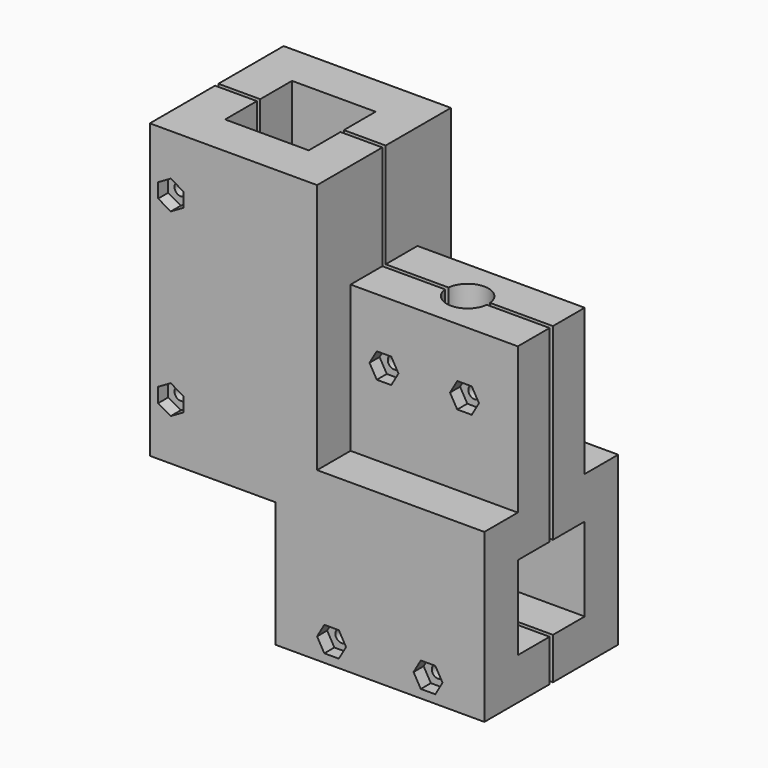
from build123d import *

# Parameters (mm, degrees)
F1_DEPTH        = 20
F2_W            = 50
F2_H            = 10
F3_DEPTH        = 10
F4_W            = 50
F4_H            = 10
F5_DEPTH        = 10
F6_W            = 50
F6_H            = 10
F7_DEPTH        = 30
F8_W            = 10
F8_H            = 10
F9_DEPTH        = 60
F10_W           = 10
F10_H           = 70
F11_DEPTH       = 30
F12_R           = 5
F13_DEPTH       = 15
F16_DEPTH       = 70
F17_T1_DEPTH    = 17.2150489639
F17_S1_T1_DEPTH = 10.5
F18_W           = 10
F18_H           = 70
F18_W_2         = 50
F18_H_2         = 10
F20_DEPTH       = 9.5
F19_W           = 10
F19_H           = 70
F19_W_2         = 50
F19_H_2         = 10
F21_DEPTH       = 9.5
F22_R           = 1.5
F23_DEPTH       = 3
F24_DEPTH       = 20
F25_R           = 1.5
F26_DEPTH       = 20
F27_R           = 1.5
F28_DEPTH       = 3
F29_DEPTH       = 10
F30_R           = 1.5
F31_DEPTH       = 10


# Not quite as in the source:
# - a fillet or chamfer that OpenCascade refuses, or shapes differently, is made with other operations: its cross-section is extruded or revolved along the edge and cut away or added


with BuildPart() as f1:
    # F0 (on Front) → F1 (new body)
    with BuildSketch(Plane.XZ):
        Polygon((-40, 89.1929870069), (-50, 89.1929870069), (-50, 19.1929870069), (0, 19.1929870069), (0, 64.1929870069), (-40, 64.1929870069), align=None)
    extrude(amount=F1_DEPTH)

    # F2 (on face) → F3 (join)
    with BuildSketch(Plane.XZ.offset(20)):
        with Locations((-25, 24.1929870069)):
            Rectangle(F2_W, F2_H)
    extrude(amount=F3_DEPTH)

    # F4 (on face) → F5 (join)
    with BuildSketch(Plane(origin=(0, 0, 0), x_dir=(-1, 0, 0), z_dir=(0, 1, 0))):
        with Locations((25, 24.1929870069)):
            Rectangle(F4_W, F4_H)
    extrude(amount=F5_DEPTH)

    # F6 (on face) → F7 (join)
    with BuildSketch(Plane(origin=(0, 0, 19.1929870069), x_dir=(1, 0, 0), z_dir=(0, 0, -1))):
        with Locations((-25, 25)):
            Rectangle(F6_W, F6_H)
        with Locations((-25, -5)):
            Rectangle(F6_W, F6_H)
    extrude(amount=F7_DEPTH)

    # F8 (on face) → F9 (join)
    with BuildSketch(Plane.XY.offset(29.1929870069)):
        with Locations((-45, 5)):
            Rectangle(F8_W, F8_H)
        with Locations((-45, -25)):
            Rectangle(F8_W, F8_H)
    extrude(amount=F9_DEPTH)

    # F10 (on face) → F11 (join)
    with BuildSketch(Plane(origin=(-50, 0, 0), x_dir=(0, -1, 0), z_dir=(-1, 0, 0))):
        with Locations((25, 54.1929870069)):
            Rectangle(F10_W, F10_H)
        with Locations((-5, 54.1929870069)):
            Rectangle(F10_W, F10_H)
    extrude(amount=F11_DEPTH)

    # F12 (on face) → F13 (cut)
    with BuildSketch(Plane.XY.offset(64.1929870069)):
        with Locations((-20, -10)):
            Circle(F12_R)
    extrude(amount=-F13_DEPTH, mode=Mode.SUBTRACT)

    # F15 (on face) + F14 (on face) → F16 (cut)
    with BuildSketch(Plane.XY.offset(64.1929870069)):
        with BuildLine():
            Line((0, -10.5), (0, -9.5))
            Line((0, -9.5), (-15.0250628145, -9.5))
            ThreePointArc((-15.0250628145, -9.5), (-15.0062696344, -9.7496861247), (-15, -10))
            ThreePointArc((-15, -10), (-15.0062696344, -10.2503138753), (-15.0250628145, -10.5))
            Line((-15.0250628145, -10.5), (0, -10.5))
        make_face()
        with BuildLine():
            Line((-15.0250628145, -9.5), (-24.9749371855, -9.5))
            ThreePointArc((-24.9749371855, -9.5), (-25, -10), (-24.9749371855, -10.5))
            Line((-24.9749371855, -10.5), (-15.0250628145, -10.5))
            ThreePointArc((-15.0250628145, -10.5), (-15.0062696344, -10.2503138753), (-15, -10))
            ThreePointArc((-15, -10), (-15.0062696344, -9.7496861247), (-15.0250628145, -9.5))
        make_face()
        with BuildLine():
            Line((-24.9749371855, -9.5), (-40, -9.5))
            Line((-40, -9.5), (-40, -10.5))
            Line((-40, -10.5), (-24.9749371855, -10.5))
            ThreePointArc((-24.9749371855, -10.5), (-25, -10), (-24.9749371855, -9.5))
        make_face()
    with BuildSketch(Plane.XY.offset(89.1929870069)):
        Polygon((-40, -10.5), (-40, -10), (-40, -9.5), (-50, -9.5), (-50, -10.5), align=None)
    extrude(amount=-F16_DEPTH, mode=Mode.SUBTRACT)

    # F17: chamfer of 3 on 1 edges, made by hand

    # F17_s2 → F17_t1 (cut)
    with BuildSketch(Plane.XZ.offset(2.7849510361)):
        Polygon((-47, 19.1929870069), (-50, 22.1929870069), (-50, 19.1929870069), align=None)
    extrude(amount=F17_T1_DEPTH, mode=Mode.SUBTRACT)

    # F17#s1: chamfer of 3 on 1 edges, made by hand

    # F17_s1_s2 → F17_s1_t1 (cut)
    with BuildSketch(Plane.XZ):
        Polygon((-50, 22.1929870069), (-47, 19.1929870069), (-50, 19.1929870069), align=None)
    extrude(amount=F17_S1_T1_DEPTH, mode=Mode.SUBTRACT)

    # F18 (on face) → F20 (join)
    with BuildSketch(Plane.XZ):
        with Locations((-75, 54.1929870069)):
            Rectangle(F18_W, F18_H)
        with Locations((-25, -5.8070129931)):
            Rectangle(F18_W_2, F18_H_2)
    extrude(amount=F20_DEPTH)

    # F19 (on face) → F21 (join)
    with BuildSketch(Plane(origin=(0, -20, 0), x_dir=(-1, 0, 0), z_dir=(0, 1, 0))):
        with Locations((75, 54.1929870069)):
            Rectangle(F19_W, F19_H)
        with Locations((25, -5.8070129931)):
            Rectangle(F19_W_2, F19_H_2)
    extrude(amount=F21_DEPTH)

    # F22 (on face) → F23 (cut)
    with BuildSketch(Plane.XZ.offset(30)):
        Polygon((-72, 77.4609361993), (-75, 79.1929870069), (-78, 77.4609361993), (-78, 73.9968345842), (-75, 72.2647837766), (-72, 73.9968345842), align=None)
        with Locations((-75, 75.7288853918)):
            Circle(F22_R, mode=Mode.SUBTRACT)
        Polygon((-72, 34.3891394296), (-75, 36.1211902372), (-78, 34.3891394296), (-78, 30.9250378145), (-75, 29.1929870069), (-72, 30.9250378145), align=None)
        with Locations((-75, 32.657088622)):
            Circle(F22_R, mode=Mode.SUBTRACT)
        Polygon((-38.2679491924, -2.8070129931), (-40, -5.8070129931), (-38.2679491924, -8.8070129931), (-34.8038475773, -8.8070129931), (-33.0717967697, -5.8070129931), (-34.8038475773, -2.8070129931), align=None)
        with Locations((-36.5358983849, -5.8070129931)):
            Circle(F22_R, mode=Mode.SUBTRACT)
        Polygon((-15.1961524227, -2.8070129931), (-16.9282032303, -5.8070129931), (-15.1961524227, -8.8070129931), (-11.7320508076, -8.8070129931), (-10, -5.8070129931), (-11.7320508076, -2.8070129931), align=None)
        with Locations((-13.4641016151, -5.8070129931)):
            Circle(F22_R, mode=Mode.SUBTRACT)
    extrude(amount=-F23_DEPTH, mode=Mode.SUBTRACT)

    # F24 (cut): faces of the model
    f24_faces = [f1.faces().sort_by_distance(p)[0] for p in [
        (-75, -30, 75.7288853918),
        (-75, -30, 32.657088622),
        (-36.5358983849, -30, -5.8070129931),
        (-13.4641016151, -30, -5.8070129931),
    ]]
    extrude(f24_faces, amount=-F24_DEPTH, mode=Mode.SUBTRACT)

    # F25 (on face) → F26 (cut)
    with BuildSketch(Plane(origin=(0, 10, 0), x_dir=(-1, 0, 0), z_dir=(0, 1, 0))):
        with Locations((75, 32.657088622)):
            Circle(F25_R)
        with Locations((75, 75.7288853918)):
            Circle(F25_R)
        with Locations((36.536, -5.8070129931)):
            Circle(F25_R)
        with Locations((13.4641016151, -5.8070129931)):
            Circle(F25_R)
    extrude(amount=-F26_DEPTH, mode=Mode.SUBTRACT)

    # F27 (on face) → F28 (cut)
    with BuildSketch(Plane.XZ.offset(20)):
        Polygon((-33.7320508076, 52.1929870069), (-35.4641016151, 49.1929870069), (-33.7320508076, 46.1929870069), (-30.2679491924, 46.1929870069), (-28.5358983849, 49.1929870069), (-30.2679491924, 52.1929870069), align=None)
        with Locations((-32, 49.1929870069)):
            Circle(F27_R, mode=Mode.SUBTRACT)
        Polygon((-14.4820508076, 52.1929870069), (-16.2141016151, 49.1929870069), (-14.4820508076, 46.1929870069), (-11.0179491924, 46.1929870069), (-9.2858983849, 49.1929870069), (-11.0179491924, 52.1929870069), align=None)
        with Locations((-12.75, 49.1929870069)):
            Circle(F27_R, mode=Mode.SUBTRACT)
    extrude(amount=-F28_DEPTH, mode=Mode.SUBTRACT)

    # F29 (cut): faces of the model
    f29_faces = [f1.faces().sort_by_distance(p)[0] for p in [
        (-32, -20, 49.1929870069),
        (-12.75, -20, 49.1929870069),
    ]]
    extrude(f29_faces, amount=-F29_DEPTH, mode=Mode.SUBTRACT)

    # F30 (on face) → F31 (cut)
    with BuildSketch(Plane(origin=(0, 0, 0), x_dir=(-1, 0, 0), z_dir=(0, 1, 0))):
        with Locations((32, 49.1929870069)):
            Circle(F30_R)
        with Locations((12.75, 49.1929870069)):
            Circle(F30_R)
    extrude(amount=-F31_DEPTH, mode=Mode.SUBTRACT)


solid = f1.part
